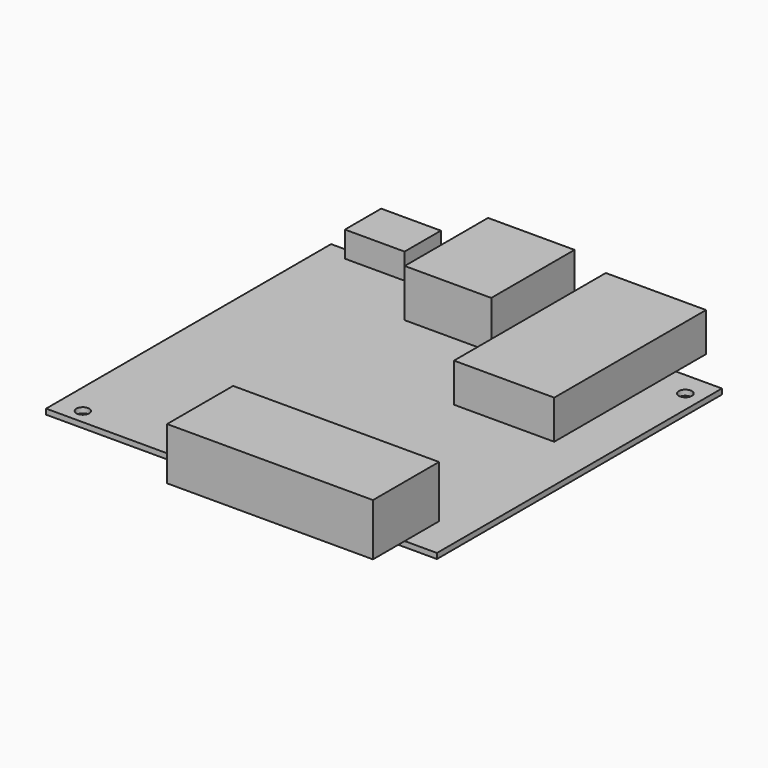
from build123d import *

# Parameters (mm, degrees)
F0_W     = 6.3
F0_H     = 16.8
F0_W_2   = 25.5
F1_DEPTH = 6.51
F0_W_3   = 6.63
F0_H_2   = 14.5
F0_W_4   = 10.82
F2_DEPTH = 8
F0_W_5   = 2.1
F0_H_3   = 10
F0_W_6   = 5.5
F3_DEPTH = 4.3
F0_W_7   = 7.18
F0_H_4   = 34.5
F0_W_8   = 6.65
F4_DEPTH = 8.75
F0_R     = 1.075
F0_R_2   = 1.1
F5_DEPTH = 0.9
F6_ANGLE = 90


# Not quite as in the source:
# - a feature of the source that left no trace in its solid (it failed there, or was rolled back) is left out


with BuildPart() as f1:
    # F0 (on Top) → F1 (new body)
    with BuildSketch(Plane.XY):
        with Locations((-39.1642118096, 33.0059126109)):
            Rectangle(F0_W, F0_H)
        with Locations((-23.2642118096, 33.0059126109)):
            Rectangle(F0_W_2, F0_H)
    extrude(amount=F1_DEPTH)


with BuildPart() as f2:
    # F0 (on Top) → F2 (new body)
    with BuildSketch(Plane.XY):
        with Locations((-39.3292118096, 11.8559126109)):
            Rectangle(F0_W_3, F0_H_2)
        with Locations((-30.6042118096, 11.8559126109)):
            Rectangle(F0_W_4, F0_H_2)
    extrude(amount=F2_DEPTH)


with BuildPart() as f3:
    # F0 (on Top) → F3 (new body)
    with BuildSketch(Plane.XY):
        with Locations((-34.9642118096, -7.3940873891)):
            Rectangle(F0_W_5, F0_H_3)
        with Locations((-38.7642118096, -7.3940873891)):
            Rectangle(F0_W_6, F0_H_3)
    extrude(amount=F3_DEPTH)


with BuildPart() as f4:
    # F0 (on Top) → F4 (new body)
    with BuildSketch(Plane.XY):
        with Locations((20.0957881904, 26.4559126109)):
            Rectangle(F0_W_7, F0_H_4)
        with Locations((27.0107881904, 26.4559126109)):
            Rectangle(F0_W_8, F0_H_4)
    extrude(amount=F4_DEPTH)


with BuildPart() as f5:
    # F0 (on Top) → F5 (new body)
    with BuildSketch(Plane.XY):
        Polygon((23.6857881904, 49.1059126109), (-36.0142118096, 49.1059126109), (-36.0142118096, 41.4059126109), (-10.5142118096, 41.4059126109), (-10.5142118096, 24.6059126109), (-36.0142118096, 24.6059126109), (-36.0142118096, 19.1059126109), (-25.1942118096, 19.1059126109), (-25.1942118096, 4.6059126109), (-36.0142118096, 4.6059126109), (-36.0142118096, -2.3940873891), (-33.9142118096, -2.3940873891), (-33.9142118096, -12.3940873891), (-36.0142118096, -12.3940873891), (-36.0142118096, -16.3940873891), (23.6857881904, -16.3940873891), (23.6857881904, 9.2059126109), (16.5057881904, 9.2059126109), (16.5057881904, 43.7059126109), (23.6857881904, 43.7059126109), align=None)
        with Locations((21.2107881904, -12.2190873891)):
            Circle(F0_R, mode=Mode.SUBTRACT)
        with Locations((-31.9142118096, 46.2559126109)):
            Circle(F0_R_2, mode=Mode.SUBTRACT)
        with Locations((20.0957881904, 26.4559126109)):
            Rectangle(F0_W_7, F0_H_4)
        with Locations((-23.2642118096, 33.0059126109)):
            Rectangle(F0_W_2, F0_H)
        with Locations((-30.6042118096, 11.8559126109)):
            Rectangle(F0_W_4, F0_H_2)
        with Locations((-34.9642118096, -7.3940873891)):
            Rectangle(F0_W_5, F0_H_3)
    extrude(amount=-F5_DEPTH)


with BuildPart() as f1_1:
    # F6: moved
    add(f1.part.rotate(Axis((-25.1942118096, 4.6059126109, 4), (0, 0, -1)), F6_ANGLE))


with BuildPart() as f2_1:
    # F6: moved
    add(f2.part.rotate(Axis((-25.1942118096, 4.6059126109, 4), (0, 0, -1)), F6_ANGLE))


with BuildPart() as f4_1:
    # F6: moved
    add(f4.part.rotate(Axis((-25.1942118096, 4.6059126109, 4), (0, 0, -1)), F6_ANGLE))


with BuildPart() as f5_1:
    # F6: moved
    add(f5.part.rotate(Axis((-25.1942118096, 4.6059126109, 4), (0, 0, -1)), F6_ANGLE))


with BuildPart() as f3_1:
    # F6: moved
    add(f3.part.rotate(Axis((-25.1942118096, 4.6059126109, 4), (0, 0, -1)), F6_ANGLE))


solid = Compound([f1_1.part, f2_1.part, f4_1.part, f5_1.part, f3_1.part])
